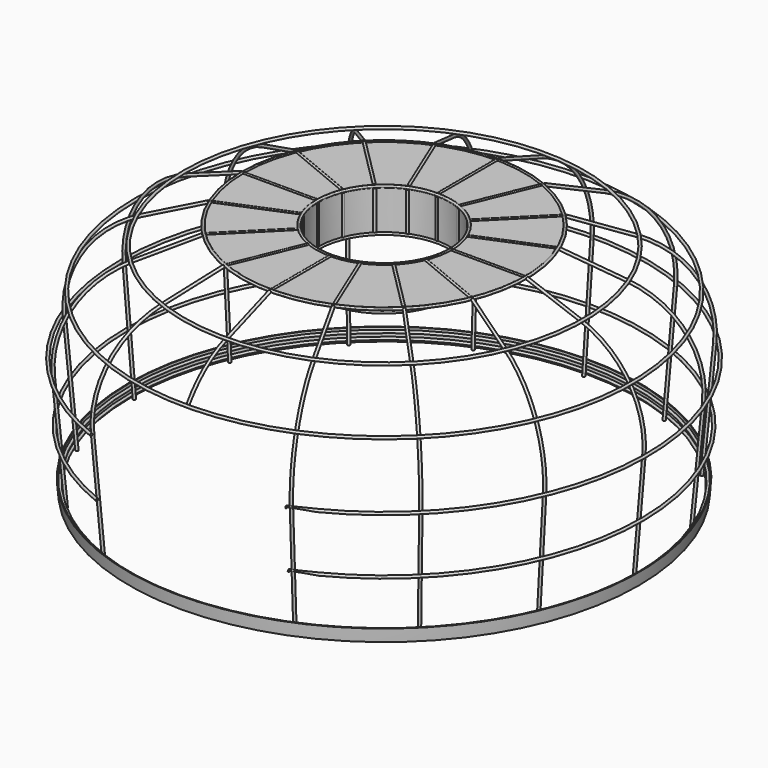
from build123d import *

# Parameters (mm, degrees)
F0_R      = 8
F4_R      = 8
F5_DEPTH  = 434
F7_R      = 8
F8_DEPTH  = 234
F9_COUNT  = 16
F11_R     = 8
F13_COUNT = 16
F14_R     = 8
F17_DEPTH = 1585.6716885149
F18_R     = 850
F18_R_2   = 400
F19_DEPTH = 2.5
F20_W     = 5
F20_H     = 250
F22_R     = 8


# Not quite as in the source:
# - an extrude ends at something that could not be found from the text; its depth is read off the source's solid


with BuildPart() as f1:
    # F0 (on Front) → F1 (revolve)
    with BuildSketch(Plane.XZ):
        with BuildLine():
            ThreePointArc((-850, 1416), (-855.6568542495, 1413.6568542495), (-858, 1408))
            ThreePointArc((-858, 1408), (-855.6568542495, 1402.3431457505), (-850, 1400))
            ThreePointArc((-850, 1400), (-844.3431457505, 1402.3431457505), (-842, 1408))
            ThreePointArc((-842, 1408), (-844.3431457505, 1413.6568542495), (-850, 1416))
        make_face()
    revolve(axis=Axis((0, 0, 700), (0, 0, 1)))


with BuildPart() as f1b:
    # F0 (on Front) → F1, piece 2 (revolve)
    with BuildSketch(Plane.XZ):
        with BuildLine():
            ThreePointArc((-392, 1408), (-394.3431457505, 1413.6568542495), (-400, 1416))
            ThreePointArc((-400, 1416), (-408, 1408), (-400, 1400))
            ThreePointArc((-400, 1400), (-394.3431457505, 1402.3431457505), (-392, 1408))
        make_face()
    revolve(axis=Axis((0, 0, 700), (0, 0, 1)))


with BuildPart() as f1c:
    # F0 (on Front) → F1, piece 3 (revolve)
    with BuildSketch(Plane.XZ):
        with Locations((-400, 1158)):
            Circle(F0_R)
    revolve(axis=Axis((0, 0, 700), (0, 0, 1)))


with BuildPart() as f5:
    # F4 (on plane+point) → F5 (new body, through all)
    with BuildSketch(Plane.YZ.offset(-408)):
        with Locations((0, 1408)):
            Circle(F4_R)
    extrude(amount=-F5_DEPTH)


with BuildPart() as f8:
    # F7 (on plane+point) → F8 (new body, through all)
    with BuildSketch(Plane.XY.offset(1166)):
        with Locations((-400, 0)):
            Circle(F7_R)
    extrude(amount=F8_DEPTH)


with BuildPart() as f9_1:
    # F9: instance of F8
    add(f8.part.rotate(Axis((0, 0, 700), (0, 0, 1)), 1 * 360 / F9_COUNT))


with BuildPart() as f9_2:
    # F9: instance of F8
    add(f8.part.rotate(Axis((0, 0, 700), (0, 0, 1)), 2 * 360 / F9_COUNT))


with BuildPart() as f9_3:
    # F9: instance of F8
    add(f8.part.rotate(Axis((0, 0, 700), (0, 0, 1)), 3 * 360 / F9_COUNT))


with BuildPart() as f9_4:
    # F9: instance of F8
    add(f8.part.rotate(Axis((0, 0, 700), (0, 0, 1)), 4 * 360 / F9_COUNT))


with BuildPart() as f9_5:
    # F9: instance of F8
    add(f8.part.rotate(Axis((0, 0, 700), (0, 0, 1)), 5 * 360 / F9_COUNT))


with BuildPart() as f9_6:
    # F9: instance of F8
    add(f8.part.rotate(Axis((0, 0, 700), (0, 0, 1)), 6 * 360 / F9_COUNT))


with BuildPart() as f9_7:
    # F9: instance of F8
    add(f8.part.rotate(Axis((0, 0, 700), (0, 0, 1)), 7 * 360 / F9_COUNT))


with BuildPart() as f9_8:
    # F9: instance of F8
    add(f8.part.rotate(Axis((0, 0, 700), (0, 0, 1)), 8 * 360 / F9_COUNT))


with BuildPart() as f9_9:
    # F9: instance of F8
    add(f8.part.rotate(Axis((0, 0, 700), (0, 0, 1)), 9 * 360 / F9_COUNT))


with BuildPart() as f9_10:
    # F9: instance of F8
    add(f8.part.rotate(Axis((0, 0, 700), (0, 0, 1)), 10 * 360 / F9_COUNT))


with BuildPart() as f9_11:
    # F9: instance of F8
    add(f8.part.rotate(Axis((0, 0, 700), (0, 0, 1)), 11 * 360 / F9_COUNT))


with BuildPart() as f9_12:
    # F9: instance of F8
    add(f8.part.rotate(Axis((0, 0, 700), (0, 0, 1)), 12 * 360 / F9_COUNT))


with BuildPart() as f9_13:
    # F9: instance of F8
    add(f8.part.rotate(Axis((0, 0, 700), (0, 0, 1)), 13 * 360 / F9_COUNT))


with BuildPart() as f9_14:
    # F9: instance of F8
    add(f8.part.rotate(Axis((0, 0, 700), (0, 0, 1)), 14 * 360 / F9_COUNT))


with BuildPart() as f9_15:
    # F9: instance of F8
    add(f8.part.rotate(Axis((0, 0, 700), (0, 0, 1)), 15 * 360 / F9_COUNT))


with BuildPart() as f9_16:
    # F9: instance of F5
    add(f5.part.rotate(Axis((0, 0, 700), (0, 0, 1)), 1 * 360 / F9_COUNT))


with BuildPart() as f9_17:
    # F9: instance of F5
    add(f5.part.rotate(Axis((0, 0, 700), (0, 0, 1)), 2 * 360 / F9_COUNT))


with BuildPart() as f9_18:
    # F9: instance of F5
    add(f5.part.rotate(Axis((0, 0, 700), (0, 0, 1)), 3 * 360 / F9_COUNT))


with BuildPart() as f9_19:
    # F9: instance of F5
    add(f5.part.rotate(Axis((0, 0, 700), (0, 0, 1)), 4 * 360 / F9_COUNT))


with BuildPart() as f9_20:
    # F9: instance of F5
    add(f5.part.rotate(Axis((0, 0, 700), (0, 0, 1)), 5 * 360 / F9_COUNT))


with BuildPart() as f9_21:
    # F9: instance of F5
    add(f5.part.rotate(Axis((0, 0, 700), (0, 0, 1)), 6 * 360 / F9_COUNT))


with BuildPart() as f9_22:
    # F9: instance of F5
    add(f5.part.rotate(Axis((0, 0, 700), (0, 0, 1)), 7 * 360 / F9_COUNT))


with BuildPart() as f9_23:
    # F9: instance of F5
    add(f5.part.rotate(Axis((0, 0, 700), (0, 0, 1)), 8 * 360 / F9_COUNT))


with BuildPart() as f9_24:
    # F9: instance of F5
    add(f5.part.rotate(Axis((0, 0, 700), (0, 0, 1)), 9 * 360 / F9_COUNT))


with BuildPart() as f9_25:
    # F9: instance of F5
    add(f5.part.rotate(Axis((0, 0, 700), (0, 0, 1)), 10 * 360 / F9_COUNT))


with BuildPart() as f9_26:
    # F9: instance of F5
    add(f5.part.rotate(Axis((0, 0, 700), (0, 0, 1)), 11 * 360 / F9_COUNT))


with BuildPart() as f9_27:
    # F9: instance of F5
    add(f5.part.rotate(Axis((0, 0, 700), (0, 0, 1)), 12 * 360 / F9_COUNT))


with BuildPart() as f9_28:
    # F9: instance of F5
    add(f5.part.rotate(Axis((0, 0, 700), (0, 0, 1)), 13 * 360 / F9_COUNT))


with BuildPart() as f9_29:
    # F9: instance of F5
    add(f5.part.rotate(Axis((0, 0, 700), (0, 0, 1)), 14 * 360 / F9_COUNT))


with BuildPart() as f9_30:
    # F9: instance of F5
    add(f5.part.rotate(Axis((0, 0, 700), (0, 0, 1)), 15 * 360 / F9_COUNT))


with BuildPart() as f12:
    # F12: sweep along a path in F0
    with BuildLine(Plane.XZ) as f12_path:
        Line((-1500, 0), (-1561.0090199234, 697.3362886642))
        ThreePointArc((-1561.0090199234, 697.3362886642), (-1472.9032293253, 1057.3949365059), (-1183.8143890683, 1289.4132604835))
        Line((-1183.8143890683, 1289.4132604835), (-858, 1408))
    # F11 (on line) → F12 (sweep)
    with BuildSketch(Plane(origin=(-11.3941852408, 0, 130.2361332502), x_dir=(0.9961946981, 0, 0.0871557427), z_dir=(-0.0871557427, 0, 0.9961946981))):
        with Locations((-1494.2920471376, 0)):
            Circle(F11_R)
    sweep(path=f12_path.line)


with BuildPart() as f13_1:
    # F13: instance of F12
    add(f12.part.rotate(Axis((0, 0, 700), (0, 0, 1)), 1 * 360 / F13_COUNT))


with BuildPart() as f13_2:
    # F13: instance of F12
    add(f12.part.rotate(Axis((0, 0, 700), (0, 0, 1)), 2 * 360 / F13_COUNT))


with BuildPart() as f13_3:
    # F13: instance of F12
    add(f12.part.rotate(Axis((0, 0, 700), (0, 0, 1)), 3 * 360 / F13_COUNT))


with BuildPart() as f13_4:
    # F13: instance of F12
    add(f12.part.rotate(Axis((0, 0, 700), (0, 0, 1)), 4 * 360 / F13_COUNT))


with BuildPart() as f13_5:
    # F13: instance of F12
    add(f12.part.rotate(Axis((0, 0, 700), (0, 0, 1)), 5 * 360 / F13_COUNT))


with BuildPart() as f13_6:
    # F13: instance of F12
    add(f12.part.rotate(Axis((0, 0, 700), (0, 0, 1)), 6 * 360 / F13_COUNT))


with BuildPart() as f13_7:
    # F13: instance of F12
    add(f12.part.rotate(Axis((0, 0, 700), (0, 0, 1)), 7 * 360 / F13_COUNT))


with BuildPart() as f13_8:
    # F13: instance of F12
    add(f12.part.rotate(Axis((0, 0, 700), (0, 0, 1)), 8 * 360 / F13_COUNT))


with BuildPart() as f13_9:
    # F13: instance of F12
    add(f12.part.rotate(Axis((0, 0, 700), (0, 0, 1)), 9 * 360 / F13_COUNT))


with BuildPart() as f13_10:
    # F13: instance of F12
    add(f12.part.rotate(Axis((0, 0, 700), (0, 0, 1)), 10 * 360 / F13_COUNT))


with BuildPart() as f13_11:
    # F13: instance of F12
    add(f12.part.rotate(Axis((0, 0, 700), (0, 0, 1)), 11 * 360 / F13_COUNT))


with BuildPart() as f13_12:
    # F13: instance of F12
    add(f12.part.rotate(Axis((0, 0, 700), (0, 0, 1)), 12 * 360 / F13_COUNT))


with BuildPart() as f13_13:
    # F13: instance of F12
    add(f12.part.rotate(Axis((0, 0, 700), (0, 0, 1)), 13 * 360 / F13_COUNT))


with BuildPart() as f13_14:
    # F13: instance of F12
    add(f12.part.rotate(Axis((0, 0, 700), (0, 0, 1)), 14 * 360 / F13_COUNT))


with BuildPart() as f13_15:
    # F13: instance of F12
    add(f12.part.rotate(Axis((0, 0, 700), (0, 0, 1)), 15 * 360 / F13_COUNT))


with BuildPart() as f15:
    # F14 (on Front) → F15 (revolve)
    with BuildSketch(Plane.XZ):
        with Locations((-1577.6706884149, 705)):
            Circle(F14_R)
    revolve(axis=Axis((0, 0, 700), (0, 0, 1)))


with BuildPart() as f15b:
    # F14 (on Front) → F15, piece 2 (revolve)
    with BuildSketch(Plane.XZ):
        with Locations((-1546.9446156253, 353)):
            Circle(F14_R)
    revolve(axis=Axis((0, 0, 700), (0, 0, 1)))


with BuildPart() as f15c:
    # F14 (on Front) → F15, piece 3 (revolve)
    with BuildSketch(Plane.XZ):
        with Locations((-1490.1645331959, 1060)):
            Circle(F14_R)
    revolve(axis=Axis((0, 0, 700), (0, 0, 1)))


with BuildPart() as f15d:
    # F14 (on Front) → F15, piece 4 (revolve)
    with BuildSketch(Plane.XZ):
        with Locations((-1201.1144993498, 1300)):
            Circle(F14_R)
    revolve(axis=Axis((0, 0, 700), (0, 0, 1)))


with BuildPart() as f17_tool:
    # F16 (on Front) → F17 (new body, through all)
    with BuildSketch(Plane.XZ):
        Polygon((-8.8809942827, 1051.525592804), (-588.3705615997, 715.5856490135), (-576.3205289841, 342.9388403893), (-9.3733714893, 9.1321375221), (9.0230377391, 9.1321375221), (576.2274861336, 342.8477346897), (585.8287811279, 715.9801721573), (9.0230377391, 1051.525592804), align=None)
    extrude(amount=F17_DEPTH)


with BuildPart() as f13_4_1:
    add(f13_4.part)

    # F17: cut by f17_tool
    add(f17_tool.part, mode=Mode.SUBTRACT)


with BuildPart() as f15_1:
    add(f15.part)

    # F17: cut by f17_tool
    add(f17_tool.part, mode=Mode.SUBTRACT)


with BuildPart() as f15b_1:
    add(f15b.part)

    # F17: cut by f17_tool
    add(f17_tool.part, mode=Mode.SUBTRACT)


with BuildPart() as f19:
    # F18 (on line) → F19 (new body, symmetric)
    with BuildSketch(Plane(origin=(0, 0, 1408), x_dir=(1, 0, 0), z_dir=(0, 0, -1))):
        Circle(F18_R)
        Circle(F18_R_2, mode=Mode.SUBTRACT)
    extrude(amount=F19_DEPTH, both=True)


with BuildPart() as f21:
    # F20 (on Front) → F21 (revolve)
    with BuildSketch(Plane.XZ):
        with Locations((-400, 1285)):
            Rectangle(F20_W, F20_H)
    revolve(axis=Axis((0, 0, 700), (0, 0, 1)))


with BuildPart() as f23:
    # F22 (on Front) → F23 (revolve)
    with BuildSketch(Plane.XZ):
        with Locations((-1517.8565415099, 20.5217914741)):
            Circle(F22_R)
    revolve(axis=Axis((0, 0, 700), (0, 0, 1)))


with BuildPart() as f23b:
    # F22 (on Front) → F23, piece 2 (revolve)
    with BuildSketch(Plane.XZ):
        with Locations((-1520.9069925061, 55.3886059073)):
            Circle(F22_R)
    revolve(axis=Axis((0, 0, 700), (0, 0, 1)))


with BuildPart() as f25:
    # F24 (on Front) → F25 (revolve)
    with BuildSketch(Plane.XZ):
        Polygon((-1529.0726495915, -0.4357787137), (-1524.091676101, 0), (-1530.6283568071, 74.7146023569), (-1535.6093302976, 74.2788236431), align=None)
    revolve(axis=Axis((0, 0, 700), (0, 0, 1)))


solid = Compound([f1.part, f1b.part, f1c.part, f5.part, f8.part, f9_1.part, f9_2.part, f9_3.part, f9_4.part, f9_5.part, f9_6.part, f9_7.part, f9_8.part, f9_9.part, f9_10.part, f9_11.part, f9_12.part, f9_13.part, f9_14.part, f9_15.part, f9_16.part, f9_17.part, f9_18.part, f9_19.part, f9_20.part, f9_21.part, f9_22.part, f9_23.part, f9_24.part, f9_25.part, f9_26.part, f9_27.part, f9_28.part, f9_29.part, f9_30.part, f12.part, f13_1.part, f13_2.part, f13_3.part, f13_5.part, f13_6.part, f13_7.part, f13_8.part, f13_9.part, f13_10.part, f13_11.part, f13_12.part, f13_13.part, f13_14.part, f13_15.part, f15c.part, f15d.part, f13_4_1.part, f15_1.part, f15b_1.part, f19.part, f21.part, f23.part, f23b.part, f25.part])
